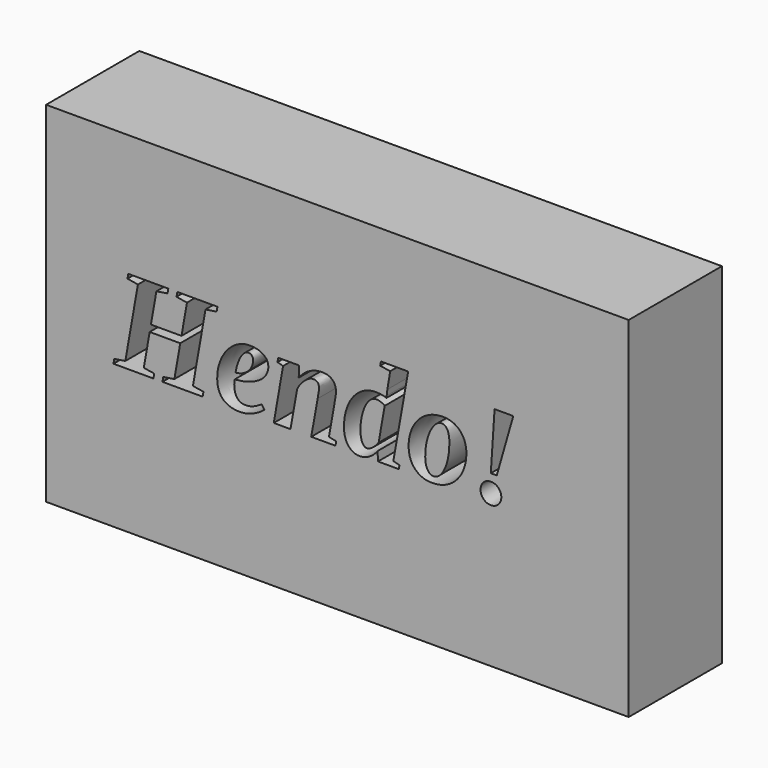
from build123d import *

# Parameters (mm, degrees)
F0_W         = 50
F0_H         = 30
F1_DEPTH     = 10
F2_TEXT_SIZE = 11.0089939549
F3_DEPTH     = 10


# Not quite as in the source:
# - Text() gives the source's letters only with a copy of the font that has no kerning and outlines rounded to 1/6400 em; it was checked with that copy


with BuildPart() as f1:
    # F0 (on Front) → F1 (new body)
    with BuildSketch(Plane.XZ):
        with Locations((15.8606082201, -0.6698413193)):
            Rectangle(F0_W, F0_H)
    extrude(amount=F1_DEPTH)

    # F2 (on face) → F3 (cut)
    with BuildSketch(Plane.XZ.offset(10)):
        with Locations((-3.2746513329, -3.3561493293)):
            Text('Hendo!', F2_TEXT_SIZE, font='Tinos', font_style=FontStyle.BOLDITALIC, text_align=(TextAlign.LEFT, TextAlign.BOTTOM))
    extrude(amount=-F3_DEPTH, mode=Mode.SUBTRACT)


solid = f1.part
